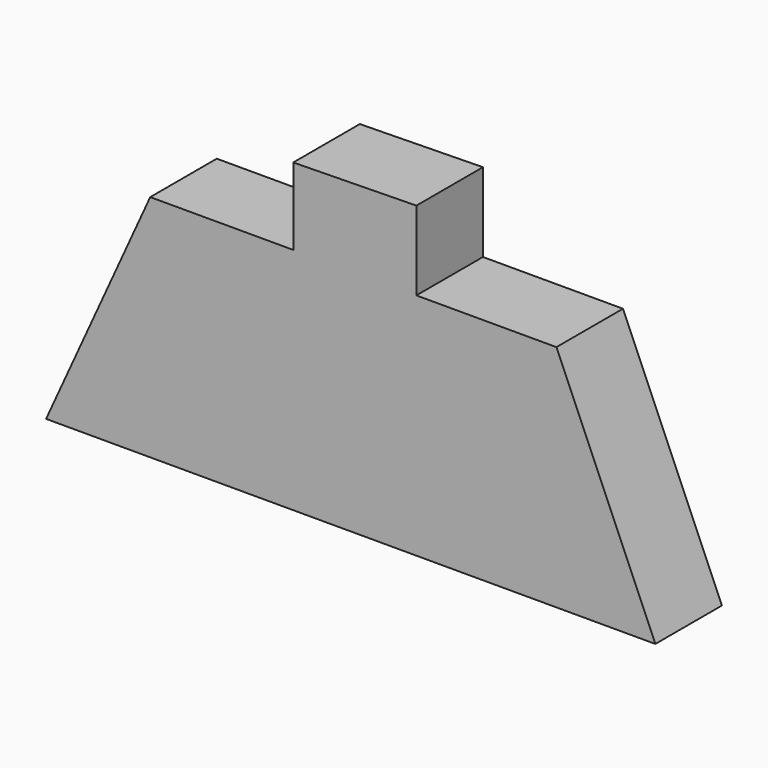
from build123d import *

# Parameters (mm, degrees)
F1_DEPTH = 2.54


# Not quite as in the source:
# - a feature names something its author has since deleted; it is built from what else it names


with BuildPart() as f1:
    # F0 (on Front) → F1 (new body)
    with BuildSketch(Plane.XZ):
        Polygon((-1.7542706408, -20.5894294426), (2.0046659093, -20.5894294426), (2.0046659093, -18.1758526358), (-1.7542706408, -18.2386604086), align=None)
        Polygon((-9.3010173015, -27.5850638216), (9.3010173015, -27.5850638216), (6.2801731089, -20.5894294426), (2.0046659093, -20.5894294426), (-1.7542706408, -20.5894294426), (-6.1211816028, -20.5894294426), align=None)
    extrude(amount=F1_DEPTH)


solid = f1.part
